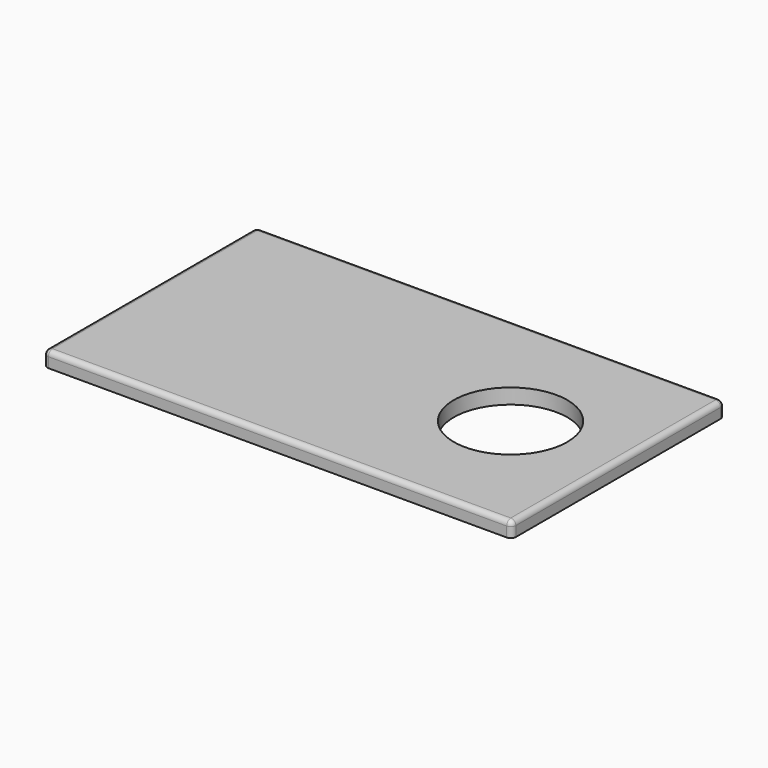
from build123d import *

# Parameters (mm, degrees)
F0_W         = 185.6
F0_H         = 105.4
F1_DEPTH     = 6
F2_R         = 22.5
F3_DEPTH     = 25
F4_R         = 2
F5_T1_DEPTH  = 9
F5_S5_W      = 2
F5_S5_H      = 2
F5_T6_DEPTH  = 2
F5_S11_W     = 2
F5_S11_H     = 2
F5_T12_DEPTH = 2
F5_S17_W     = 2
F5_S17_H     = 2
F5_T18_DEPTH = 2
F5_S23_W     = 2
F5_S23_H     = 2
F5_T24_DEPTH = 2


# Not quite as in the source:
# - a fillet or chamfer that OpenCascade refuses, or shapes differently, is made with other operations: its cross-section is extruded or revolved along the edge and cut away or added


with BuildPart() as f1:
    # F0 (on Top) → F1 (new body)
    with BuildSketch(Plane.XY):
        Rectangle(F0_W, F0_H)
    extrude(amount=F1_DEPTH)

    # F2 (on face) → F3 (cut)
    with BuildSketch(Plane.XY.offset(6)):
        with Locations((50.1459216796, 0)):
            Circle(F2_R)
    extrude(amount=-F3_DEPTH, mode=Mode.SUBTRACT)

    # F4
    f4_edges = [f1.edges().sort_by_distance(p)[0] for p in [
        (0, -52.7, 6),
        (92.8, 0, 6),
        (0, 52.7, 6),
        (-92.8, 0, 6),
    ]]
    fillet(f4_edges, radius=F4_R)

    # F5: fillet of radius 2 on 4 edges, made by hand

    # F5_s2 → F5_t1 (cut)
    with BuildSketch(Plane.XY.offset(-5)):
        with BuildLine():
            ThreePointArc((92.8, -50.7), (92.2142135624, -52.1142135624), (90.8, -52.7))
            Line((90.8, -52.7), (92.8, -52.7))
            Line((92.8, -52.7), (92.8, -50.7))
        make_face()
        with BuildLine():
            ThreePointArc((92.8, 50.7), (92.2142135624, 52.1142135624), (90.8, 52.7))
            Line((90.8, 52.7), (92.8, 52.7))
            Line((92.8, 52.7), (92.8, 50.7))
        make_face()
        with BuildLine():
            ThreePointArc((-90.8, 52.7), (-92.2142135624, 52.1142135624), (-92.8, 50.7))
            Line((-92.8, 50.7), (-92.8, 52.7))
            Line((-92.8, 52.7), (-90.8, 52.7))
        make_face()
        with BuildLine():
            ThreePointArc((-90.8, -52.7), (-92.2142135624, -52.1142135624), (-92.8, -50.7))
            Line((-92.8, -50.7), (-92.8, -52.7))
            Line((-92.8, -52.7), (-90.8, -52.7))
        make_face()
    extrude(amount=F5_T1_DEPTH, mode=Mode.SUBTRACT)


with BuildPart() as f5_tool4:
    # F5_s5 → F5_t6 (new body)
    with BuildSketch(Plane.XZ.offset(50.7)):
        with Locations((-91.8, 5)):
            Rectangle(F5_S5_W, F5_S5_H)
    extrude(amount=F5_T6_DEPTH)

    # F5_s7 → F5_t8 (revolve, cut)
    with BuildSketch(Plane(origin=(-90.8, -50.7, 4), x_dir=(0.7071067812, 0, -0.7071067812), z_dir=(-0.7071067812, 0, -0.7071067812))):
        with BuildLine():
            ThreePointArc((0, -2), (2, 0), (0, 2))
            Line((0, 2), (0, -2))
        make_face()
    revolve(axis=Axis((-90.8, -50.7, 4), (0, -1, 0)), mode=Mode.SUBTRACT)


with BuildPart() as f1_1:
    add(f1.part)

    # F5_t3: cut F5_tool4
    add(f5_tool4.part, mode=Mode.SUBTRACT)


with BuildPart() as f5_tool10:
    # F5_s11 → F5_t12 (new body)
    with BuildSketch(Plane.XZ.offset(-50.7)):
        with Locations((-91.8, 5)):
            Rectangle(F5_S11_W, F5_S11_H)
    extrude(amount=-F5_T12_DEPTH)

    # F5_s13 → F5_t14 (revolve, cut)
    with BuildSketch(Plane(origin=(-90.8, 50.7, 4), x_dir=(0.7071067812, 0, -0.7071067812), z_dir=(0.7071067812, 0, 0.7071067812))):
        with BuildLine():
            ThreePointArc((0, -2), (2, 0), (0, 2))
            Line((0, 2), (0, -2))
        make_face()
    revolve(axis=Axis((-90.8, 50.7, 4), (0, 1, 0)), mode=Mode.SUBTRACT)


with BuildPart() as f1_2:
    add(f1_1.part)

    # F5_t9: cut F5_tool10
    add(f5_tool10.part, mode=Mode.SUBTRACT)


with BuildPart() as f5_tool16:
    # F5_s17 → F5_t18 (new body)
    with BuildSketch(Plane.YZ.offset(90.8)):
        with Locations((51.7, 5)):
            Rectangle(F5_S17_W, F5_S17_H)
    extrude(amount=F5_T18_DEPTH)

    # F5_s19 → F5_t20 (revolve, cut)
    with BuildSketch(Plane(origin=(90.8, 50.7, 4), x_dir=(0, -0.7071067812, -0.7071067812), z_dir=(0, -0.7071067812, 0.7071067812))):
        with BuildLine():
            ThreePointArc((0, -2), (2, 0), (0, 2))
            Line((0, 2), (0, -2))
        make_face()
    revolve(axis=Axis((90.8, 50.7, 4), (1, 0, 0)), mode=Mode.SUBTRACT)


with BuildPart() as f1_3:
    add(f1_2.part)

    # F5_t15: cut F5_tool16
    add(f5_tool16.part, mode=Mode.SUBTRACT)


with BuildPart() as f5_tool22:
    # F5_s23 → F5_t24 (new body)
    with BuildSketch(Plane.YZ.offset(90.8)):
        with Locations((-51.7, 5)):
            Rectangle(F5_S23_W, F5_S23_H)
    extrude(amount=F5_T24_DEPTH)

    # F5_s25 → F5_t26 (revolve, cut)
    with BuildSketch(Plane(origin=(90.8, -50.7, 4), x_dir=(0, 0.7071067812, -0.7071067812), z_dir=(0, -0.7071067812, -0.7071067812))):
        with BuildLine():
            ThreePointArc((0, -2), (2, 0), (0, 2))
            Line((0, 2), (0, -2))
        make_face()
    revolve(axis=Axis((90.8, -50.7, 4), (1, 0, 0)), mode=Mode.SUBTRACT)


with BuildPart() as f1_4:
    add(f1_3.part)

    # F5_t21: cut F5_tool22
    add(f5_tool22.part, mode=Mode.SUBTRACT)


solid = f1_4.part
